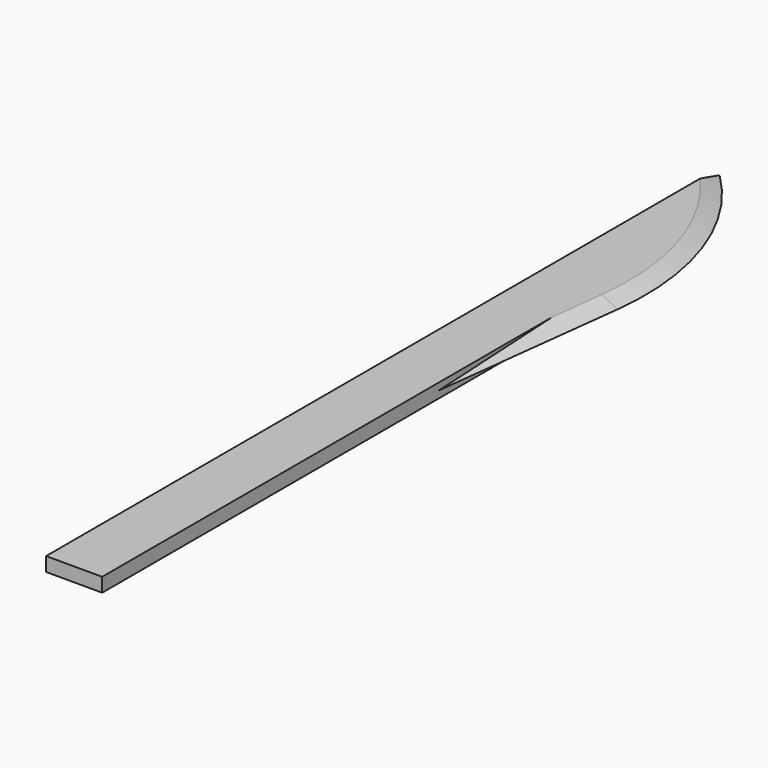
from build123d import *

# Parameters (mm, degrees)
F1_DEPTH = 1.27
F2_SIZE2 = 1.524
F2_SIZE  = 0.635
F3_SIZE2 = 0.63499
F3_SIZE  = 1.52399


# Not quite as in the source:
# - a fillet or chamfer is up to 0.001 mm smaller than in the source, because OpenCascade refuses the exact size


with BuildPart() as f1:
    # F0 (on Top) → F1 (new body)
    with BuildSketch(Plane.XY):
        with BuildLine():
            Line((-36.8330654015, 25.4), (-36.8330654015, 0))
            Line((-36.8330654015, 0), (-31.7530654015, 0))
            Line((-31.7530654015, 0), (-31.7530654015, 25.4))
            Line((-31.7530654015, 25.4), (-31.7530654015, 38.1))
            Line((-31.7530654015, 38.1), (-29.6483766288, 55.6414723396))
            ThreePointArc((-29.6483766288, 55.6414723396), (-30.8576350362, 66.7535648315), (-36.8330654015, 76.2))
            Line((-36.8330654015, 76.2), (-36.8330654015, 25.4))
        make_face()
    extrude(amount=F1_DEPTH)

    # F2
    f2_edges = [f1.edges().sort_by_distance(p)[0] for p in [
        (-30.857635, 66.753565, 0),
    ]]
    f2_side = f1.faces().sort_by_distance((-30.857635, 66.753565, 0.635))[0]
    chamfer(f2_edges, length=F2_SIZE, length2=F2_SIZE2, reference=f2_side)

    # F3 (size 1.524 and 0.635 in the source; OpenCascade refuses exactly that, so slightly less here)
    f3_edges = [f1.edges().sort_by_distance(p)[0] for p in [
        (-30.857635, 66.753565, 1.27),
    ]]
    f3_side = f1.faces().sort_by_distance((-33.993145, 38.475909, 1.27))[0]
    chamfer(f3_edges, length=F3_SIZE, length2=F3_SIZE2, reference=f3_side)


solid = f1.part
